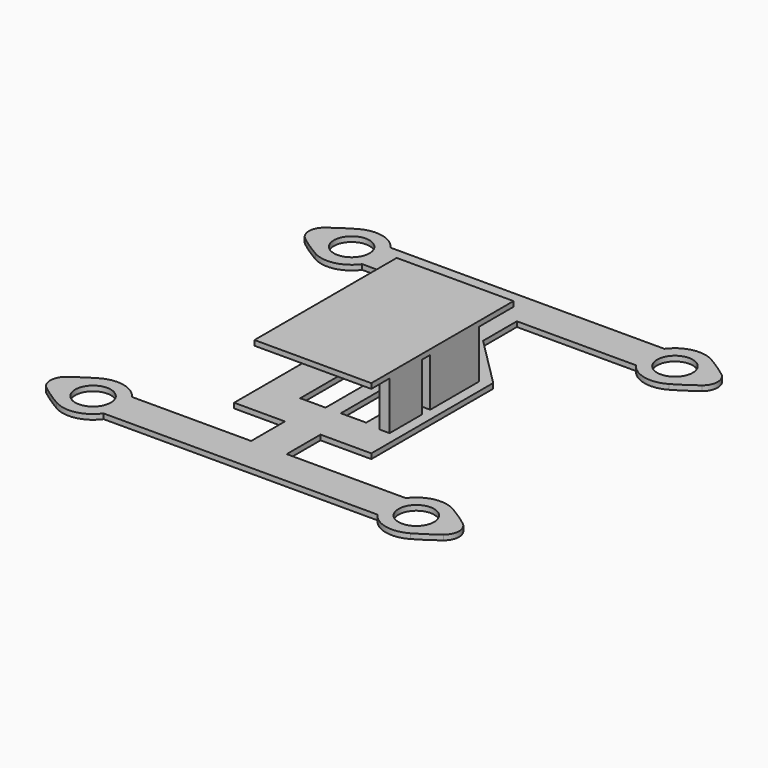
from build123d import *

# Parameters (mm, degrees)
F0_R     = 3.5
F0_W     = 5
F0_H     = 25
F1_DEPTH = 1
F2_W     = 2
F2_H     = 12
F2_H_2   = 8
F3_DEPTH = 9.5
F4_W     = 23
F4_H     = 35
F5_DEPTH = 1


# Not quite as in the source:
# - ends of sketch curves that miss each other by under 0.0002 mm in the source are joined


with BuildPart() as f1:
    # F0 (on Top) → F1 (new body)
    with BuildSketch(Plane.XY):
        with BuildLine():
            ThreePointArc((-26.946407646, 28.3198056199), (-26.1083961747, 29.9813798822), (-25.8198051534, 31.8198051534))
            ThreePointArc((-25.8198051534, 31.8198051534), (-26.1083962627, 33.6582306979), (-26.946407981, 35.3198051534))
            ThreePointArc((-26.946407981, 35.3198051534), (-30.5562239326, 37.6852431164), (-34.8198051534, 37.0159575761))
            ThreePointArc((-34.8198051534, 37.0159575761), (-37.8198051534, 31.8198051534), (-34.8198051534, 26.6236527307))
            ThreePointArc((-34.8198051534, 26.6236527307), (-30.5562236518, 25.9543672508), (-26.946407646, 28.3198056199))
        make_face()
        with Locations((-31.8198051534, 31.8198051534)):
            Circle(F0_R, mode=Mode.SUBTRACT)
        with BuildLine():
            ThreePointArc((-26.946407981, 35.3198051534), (-26.1083962627, 33.6582306979), (-25.8198051534, 31.8198051534))
            ThreePointArc((-25.8198051534, 31.8198051534), (-26.1083961747, 29.9813798822), (-26.946407646, 28.3198056199))
            Line((-26.946407646, 28.3198056199), (-3.5, 28.3198058605))
            Line((-3.5, 28.3198058605), (-3.5, 20))
            Line((-3.5, 20), (-13.5, 10))
            Line((-13.5, 10), (-13.5, -20))
            Line((-13.5, -20), (-3.5, -20))
            Line((-3.5, -20), (-3.5, -28.3198058605))
            Line((-3.5, -28.3198058605), (-26.946407981, -28.3198058605))
            ThreePointArc((-26.946407981, -28.3198058605), (-26.1083961747, -29.9813798822), (-25.8198051534, -31.8198051534))
            ThreePointArc((-25.8198051534, -31.8198051534), (-26.1083962627, -33.6582306979), (-26.946407981, -35.3198051534))
            Line((-26.946407981, -35.3198051534), (26.946407981, -35.3198051534))
            ThreePointArc((26.946407981, -35.3198051534), (25.8198051534, -31.8198054406), (26.946407646, -28.3198056199))
            Line((26.946407646, -28.3198056199), (3.5, -28.3198058605))
            Line((3.5, -28.3198058605), (3.5, -20))
            Line((3.5, -20), (13.5, -20))
            Line((13.5, -20), (13.5, 10))
            Line((13.5, 10), (3.5, 20))
            Line((3.5, 20), (3.5, 28.3198058605))
            Line((3.5, 28.3198058605), (26.946407981, 28.3198058605))
            ThreePointArc((26.946407981, 28.3198058605), (25.8198051534, 31.8198054406), (26.946407981, 35.3198051534))
            Line((26.946407981, 35.3198051534), (-26.946407981, 35.3198051534))
        make_face()
        with Locations((-4, 0)):
            Rectangle(F0_W, F0_H, mode=Mode.SUBTRACT)
        with Locations((4, 0)):
            Rectangle(F0_W, F0_H, mode=Mode.SUBTRACT)
        with BuildLine():
            ThreePointArc((-34.8198051534, 26.6236527307), (-37.8198051534, 31.8198051534), (-34.8198051534, 37.0159575761))
            ThreePointArc((-34.8198051534, 37.0159575761), (-36.975362446, 35.6785640663), (-39.041812183, 34.2072265368))
            ThreePointArc((-39.041812183, 34.2072265368), (-40.2251616558, 31.8198051534), (-39.041812183, 29.43238377))
            ThreePointArc((-39.041812183, 29.43238377), (-36.975362446, 27.9610462405), (-34.8198051534, 26.6236527307))
        make_face()
        with BuildLine():
            ThreePointArc((34.8198051534, 37.0159575761), (30.5562239326, 37.6852431164), (26.946407981, 35.3198051534))
            ThreePointArc((26.946407981, 35.3198051534), (25.8198051534, 31.8198054406), (26.946407646, 28.3198056199))
            ThreePointArc((26.946407646, 28.3198056199), (30.5562236518, 25.9543672508), (34.8198051534, 26.6236527307))
            ThreePointArc((34.8198051534, 26.6236527307), (37.0159575761, 28.8198051534), (37.8198051534, 31.8198051534))
            ThreePointArc((37.8198051534, 31.8198051534), (37.0159575761, 34.8198051534), (34.8198051534, 37.0159575761))
        make_face()
        with Locations((31.8198051534, 31.8198051534)):
            Circle(F0_R, mode=Mode.SUBTRACT)
        with BuildLine():
            ThreePointArc((39.041812183, 34.2072265368), (36.975362446, 35.6785640663), (34.8198051534, 37.0159575761))
            ThreePointArc((34.8198051534, 37.0159575761), (37.0159575761, 34.8198051534), (37.8198051534, 31.8198051534))
            ThreePointArc((37.8198051534, 31.8198051534), (37.0159575761, 28.8198051534), (34.8198051534, 26.6236527307))
            ThreePointArc((34.8198051534, 26.6236527307), (36.975362446, 27.9610462405), (39.041812183, 29.43238377))
            ThreePointArc((39.041812183, 29.43238377), (40.2251616558, 31.8198051534), (39.041812183, 34.2072265368))
        make_face()
        with BuildLine():
            ThreePointArc((-25.8198051534, -31.8198051534), (-26.1083961747, -29.9813798822), (-26.946407646, -28.3198056199))
            ThreePointArc((-26.946407646, -28.3198056199), (-30.5562236518, -25.9543672508), (-34.8198051534, -26.6236527307))
            ThreePointArc((-34.8198051534, -26.6236527307), (-37.8198051534, -31.8198051534), (-34.8198051534, -37.0159575761))
            ThreePointArc((-34.8198051534, -37.0159575761), (-30.5562239326, -37.6852431164), (-26.946407981, -35.3198051534))
            ThreePointArc((-26.946407981, -35.3198051534), (-26.1083962627, -33.6582306979), (-25.8198051534, -31.8198051534))
        make_face()
        with Locations((-31.8198051534, -31.8198051534)):
            Circle(F0_R, mode=Mode.SUBTRACT)
        with BuildLine():
            ThreePointArc((-34.8198051534, -37.0159575761), (-37.8198051534, -31.8198051534), (-34.8198051534, -26.6236527307))
            ThreePointArc((-34.8198051534, -26.6236527307), (-36.975362446, -27.9610462405), (-39.041812183, -29.43238377))
            ThreePointArc((-39.041812183, -29.43238377), (-40.2251616558, -31.8198051534), (-39.041812183, -34.2072265368))
            ThreePointArc((-39.041812183, -34.2072265368), (-36.975362446, -35.6785640663), (-34.8198051534, -37.0159575761))
        make_face()
        with BuildLine():
            ThreePointArc((34.8198051534, -26.6236527307), (30.5562236518, -25.9543672508), (26.946407646, -28.3198056199))
            ThreePointArc((26.946407646, -28.3198056199), (25.8198051534, -31.8198054406), (26.946407981, -35.3198051534))
            ThreePointArc((26.946407981, -35.3198051534), (30.5562239326, -37.6852431164), (34.8198051534, -37.0159575761))
            ThreePointArc((34.8198051534, -37.0159575761), (37.0159575761, -34.8198051534), (37.8198051534, -31.8198051534))
            ThreePointArc((37.8198051534, -31.8198051534), (37.0159575761, -28.8198051534), (34.8198051534, -26.6236527307))
        make_face()
        with Locations((31.8198051534, -31.8198051534)):
            Circle(F0_R, mode=Mode.SUBTRACT)
        with BuildLine():
            ThreePointArc((39.041812183, -29.43238377), (36.975362446, -27.9610462405), (34.8198051534, -26.6236527307))
            ThreePointArc((34.8198051534, -26.6236527307), (37.0159575761, -28.8198051534), (37.8198051534, -31.8198051534))
            ThreePointArc((37.8198051534, -31.8198051534), (37.0159575761, -34.8198051534), (34.8198051534, -37.0159575761))
            ThreePointArc((34.8198051534, -37.0159575761), (36.975362446, -35.6785640663), (39.041812183, -34.2072265368))
            ThreePointArc((39.041812183, -34.2072265368), (40.2251616558, -31.8198051534), (39.041812183, -29.43238377))
        make_face()
    extrude(amount=F1_DEPTH)

    # F2 (on face) → F3 (join)
    with BuildSketch(Plane.XY.offset(1)):
        with Locations((-10.5, 3)):
            Rectangle(F2_W, F2_H)
        with Locations((10.5, 3)):
            Rectangle(F2_W, F2_H)
        with Locations((10.5, -9)):
            Rectangle(F2_W, F2_H_2)
    extrude(amount=F3_DEPTH)

    # F4 (on face) → F5 (join)
    with BuildSketch(Plane.XY.offset(10.5)):
        Rectangle(F4_W, F4_H)
    extrude(amount=F5_DEPTH)


solid = f1.part
